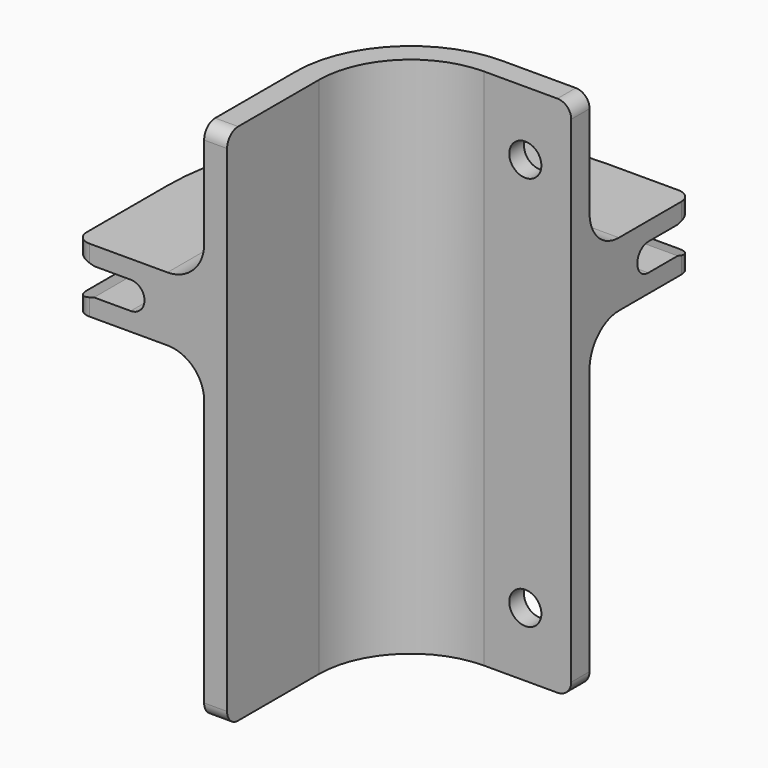
from build123d import *

# Parameters (mm, degrees)
F1_DEPTH  = 40
F3_DEPTH  = 6.5
F4_DEPTH  = 14
F5_R      = 3.5
F5_R_2    = 1.75
F6_DEPTH  = 0.5
F7_DEPTH  = 25
F8_DEPTH  = 17
F9_R      = 1.75
F10_DEPTH = 3
F9_R_2    = 3.5
F11_DEPTH = 0.5
F12_W     = 12.5
F12_H     = 3
F13_DEPTH = 6.5
F12_H_2   = 2
F14_DEPTH = 14
F15_ANGLE = 90
F16_R     = 4
F17_SIZE2 = 2
F17_SIZE  = 0.6
F18_SIZE2 = 0.6
F18_SIZE  = 2
F19_R     = 1.49999


# Not quite as in the source:
# - a fillet or chamfer is up to 0.001 mm smaller than in the source, because OpenCascade refuses the exact size


with BuildPart() as f1:
    # F0 (on Top) → F1 (new body)
    with BuildSketch(Plane.XY):
        with BuildLine():
            ThreePointArc((-10, 0), (-7.0710678119, 7.0710678119), (0, 10))
            Line((0, 10), (9.5, 10))
            Line((9.5, 10), (9.5, 12.5))
            Line((9.5, 12.5), (0, 12.5))
            ThreePointArc((0, 12.5), (-8.8388347648, 8.8388347648), (-12.5, 0))
            Line((-12.5, 0), (-12.5, -12.5))
            Line((-12.5, -12.5), (-10, -12.5))
            Line((-10, -12.5), (-10, 0))
        make_face()
    extrude(amount=F1_DEPTH)

    # F2 (on face) → F3 (join)
    with BuildSketch(Plane(origin=(0, 12.5, 0), x_dir=(-1, 0, 0), z_dir=(0, 1, 0))):
        Polygon((-5.7388888672, 22.5), (-9.5, 22.5), (-9.5, 19.5), (-5.7327155955, 19.5), (0, 19.5), (0, 22.5), align=None)
    extrude(amount=F3_DEPTH)

    # F2 (on face) → F4 (join)
    with BuildSketch(Plane(origin=(0, 12.5, 0), x_dir=(-1, 0, 0), z_dir=(0, 1, 0))):
        Polygon((-5.7188421488, 24.5), (-9.5, 24.5), (-9.5, 22.5), (-5.7388888672, 22.5), (0, 22.5), (0, 24.5), align=None)
        Polygon((-5.7327155955, 19.5), (-9.5, 19.5), (-9.5, 17.5), (-5.7445626465, 17.5), (0, 17.5), (0, 19.5), align=None)
    extrude(amount=F4_DEPTH)

    # F5 (on face) → F6 (cut)
    with BuildSketch(Plane(origin=(0, 12.5, 0), x_dir=(-1, 0, 0), z_dir=(0, 1, 0))):
        with Locations((-4.5, 33)):
            Circle(F5_R)
        with Locations((-4.5, 33)):
            Circle(F5_R_2, mode=Mode.SUBTRACT)
    extrude(amount=-F6_DEPTH, mode=Mode.SUBTRACT)

    # F5 (on face) → F7 (cut)
    with BuildSketch(Plane(origin=(0, 12.5, 0), x_dir=(-1, 0, 0), z_dir=(0, 1, 0))):
        with Locations((-4.5, 33)):
            Circle(F5_R_2)
    extrude(amount=-F7_DEPTH, mode=Mode.SUBTRACT)

    # F8 (add): a face of the model
    f8_faces = [f1.faces().sort_by_distance(p)[0] for p in [
        (-7.3065460487, 7.3065460487, 0),
    ]]
    extrude(f8_faces, amount=F8_DEPTH)

    # F9 (on face) → F10 (cut)
    with BuildSketch(Plane(origin=(0, 12.5, 0), x_dir=(-1, 0, 0), z_dir=(0, 1, 0))):
        with Locations((-4.5, -10)):
            Circle(F9_R)
    extrude(amount=-F10_DEPTH, mode=Mode.SUBTRACT)

    # F9 (on face) → F11 (cut)
    with BuildSketch(Plane(origin=(0, 12.5, 0), x_dir=(-1, 0, 0), z_dir=(0, 1, 0))):
        with Locations((-4.5, -10)):
            Circle(F9_R_2)
        with Locations((-4.5, -10)):
            Circle(F9_R, mode=Mode.SUBTRACT)
    extrude(amount=-F11_DEPTH, mode=Mode.SUBTRACT)

    # F12 (on face) → F13 (join)
    with BuildSketch(Plane(origin=(-12.5, 0, 0), x_dir=(0, -1, 0), z_dir=(-1, 0, 0))):
        with Locations((6.25, 21)):
            Rectangle(F12_W, F12_H)
    extrude(amount=F13_DEPTH)

    # F12 (on face) → F14 (join)
    with BuildSketch(Plane(origin=(-12.5, 0, 0), x_dir=(0, -1, 0), z_dir=(-1, 0, 0))):
        with Locations((6.25, 23.5)):
            Rectangle(F12_W, F12_H_2)
        with Locations((6.25, 18.5)):
            Rectangle(F12_W, F12_H_2)
    extrude(amount=F14_DEPTH)

    # F14_face (on face) → F15 (revolve)
    with BuildSketch(Plane(origin=(-18.5314569536, 0, 21), x_dir=(-1, 0, 0), z_dir=(0, 1, 0))):
        Polygon((7.9685430464, -1.5), (0.4685430464, -1.5), (0.4685430464, 1.5), (7.9685430464, 1.5), (7.9685430464, 3.5), (-6.0314569536, 3.5), (-6.0314569536, -3.5), (7.9685430464, -3.5), align=None)
    revolve(axis=Axis((0, 0, 0), (0, 0, -1)), revolution_arc=F15_ANGLE)

    # F16
    f16_edges = [f1.edges().sort_by_distance(p)[0] for p in [
        (-8.838835, 8.838835, 17.5),
        (-8.838835, 8.838835, 24.5),
    ]]
    fillet(f16_edges, radius=F16_R)

    # F17
    f17_edges = [f1.edges().sort_by_distance(p)[0] for p in [
        (-26.5, -6.25, 19.5),
    ]]
    f17_side = f1.faces().sort_by_distance((-26.5, -6.25, 18.5))[0]
    chamfer(f17_edges, length=F17_SIZE, length2=F17_SIZE2, reference=f17_side)

    # F18
    f18_edges = [f1.edges().sort_by_distance(p)[0] for p in [
        (-26.5, -6.25, 22.5),
    ]]
    f18_side = f1.faces().sort_by_distance((-19.530754, -6.25, 22.5))[0]
    chamfer(f18_edges, length=F18_SIZE, length2=F18_SIZE2, reference=f18_side)

    # F19 (radius 1.5 in the source; OpenCascade refuses exactly that, so slightly less here)
    f19_edges = [f1.edges().sort_by_distance(p)[0] for p in [
        (-13.435029, 13.435029, 19.5),
        (-13.435029, 13.435029, 22.5),
        (9.5, 26.5, 23.8),
        (9.5, 26.5, 18.2),
        (-26.5, -12.5, 18.2),
        (-26.5, -12.5, 23.8),
        (-11.25, -12.5, 40),
        (9.5, 11.25, 40),
        (9.5, 11.25, -17),
        (-11.25, -12.5, -17),
    ]]
    fillet(f19_edges, radius=F19_R)


solid = f1.part
